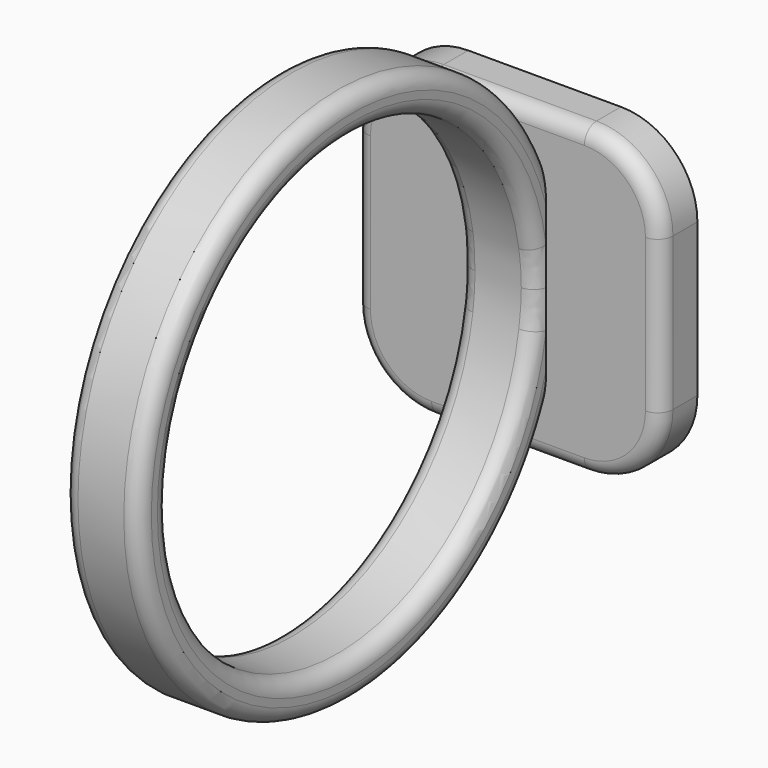
from build123d import *

# Parameters (mm, degrees)
F0_W         = 20
F0_H         = 20
F1_DEPTH     = 3
F2_R         = 17.5
F2_R_2       = 15
F3_DEPTH     = 2.5
F4_R         = 1
F5_T1_DEPTH  = 15.5
F5_T4_ANGLE  = 90
F5_T6_ANGLE  = 90
F5_T8_ANGLE  = 90
F5_T10_ANGLE = 90


# Not quite as in the source:
# - a fillet or chamfer that OpenCascade refuses, or shapes differently, is made with other operations: its cross-section is extruded or revolved along the edge and cut away or added


with BuildPart() as f1:
    # F0 (on Front) → F1 (new body)
    with BuildSketch(Plane.XZ):
        Rectangle(F0_W, F0_H)
    extrude(amount=F1_DEPTH)

    # F2 (on Right) → F3 (join, symmetric)
    with BuildSketch(Plane.YZ):
        with Locations((-18.8078675419, 0)):
            Circle(F2_R)
        with Locations((-18.8078675419, 0)):
            Circle(F2_R_2, mode=Mode.SUBTRACT)
    extrude(amount=F3_DEPTH, both=True)

    # F4 (call 1 of 5: OpenCascade refuses the feature's edges together)
    f4_edges = [f1.edges().sort_by_distance(p)[0] for p in [
        (2.5, -36.307868, 0),
    ]]
    fillet(f4_edges, radius=F4_R)

    # F4#2 (call 2 of 5)
    f4_2_edges = [f1.edges().sort_by_distance(p)[0] for p in [
        (-2.5, -36.307868, 0),
    ]]
    fillet(f4_2_edges, radius=F4_R)

    # F4#3 (call 3 of 5)
    f4_3_edges = [f1.edges().sort_by_distance(p)[0] for p in [
        (-2.5, -33.807868, 0),
    ]]
    fillet(f4_3_edges, radius=F4_R)

    # F4#4 (call 4 of 5)
    f4_4_edges = [f1.edges().sort_by_distance(p)[0] for p in [
        (2.5, -33.807868, 0),
    ]]
    fillet(f4_4_edges, radius=F4_R)

    # F4#5 (call 5 of 5)
    f4_5_edges = [f1.edges().sort_by_distance(p)[0] for p in [
        (10, -3, 0),
        (0, -3, 10),
        (-10, -3, 0),
        (0, -3, -10),
    ]]
    fillet(f4_5_edges, radius=F4_R)

    # F5: fillet of radius 5 on 4 edges, made by hand

    # F5_s2 → F5_t1 (cut)
    with BuildSketch(Plane.XZ.offset(-12.5)):
        with BuildLine():
            ThreePointArc((-5, 10), (-8.5355339059, 8.5355339059), (-10, 5))
            Line((-10, 5), (-10, 10))
            Line((-10, 10), (-5, 10))
        make_face()
        with BuildLine():
            ThreePointArc((-5, -10), (-8.5355339059, -8.5355339059), (-10, -5))
            Line((-10, -5), (-10, -10))
            Line((-10, -10), (-5, -10))
        make_face()
        with BuildLine():
            ThreePointArc((10, 5), (8.5355339059, 8.5355339059), (5, 10))
            Line((5, 10), (10, 10))
            Line((10, 10), (10, 5))
        make_face()
        with BuildLine():
            ThreePointArc((10, -5), (8.5355339059, -8.5355339059), (5, -10))
            Line((5, -10), (10, -10))
            Line((10, -10), (10, -5))
        make_face()
    extrude(amount=F5_T1_DEPTH, mode=Mode.SUBTRACT)

    # F5_s3 → F5_t4 (revolve, cut)
    with BuildSketch(Plane.YZ.offset(5)):
        with BuildLine():
            ThreePointArc((-3, -9), (-2.7071067812, -9.7071067812), (-2, -10))
            Line((-2, -10), (-3, -10))
            Line((-3, -10), (-3, -9))
        make_face()
    revolve(axis=Axis((5, -3, -5), (0, -1, 0)), revolution_arc=F5_T4_ANGLE, mode=Mode.SUBTRACT)

    # F5_s5 → F5_t6 (revolve, cut)
    with BuildSketch(Plane.XY.offset(5)):
        with BuildLine():
            ThreePointArc((9, -3), (9.7071067812, -2.7071067812), (10, -2))
            Line((10, -2), (10, -3))
            Line((10, -3), (9, -3))
        make_face()
    revolve(axis=Axis((5, -3, 5), (0, -1, 0)), revolution_arc=F5_T6_ANGLE, mode=Mode.SUBTRACT)

    # F5_s7 → F5_t8 (revolve, cut)
    with BuildSketch(Plane.XY.offset(-5)):
        with BuildLine():
            ThreePointArc((-9, -3), (-9.7071067812, -2.7071067812), (-10, -2))
            Line((-10, -2), (-10, -3))
            Line((-10, -3), (-9, -3))
        make_face()
    revolve(axis=Axis((-5, -3, -5), (0, -1, 0)), revolution_arc=F5_T8_ANGLE, mode=Mode.SUBTRACT)

    # F5_s9 → F5_t10 (revolve, cut)
    with BuildSketch(Plane.YZ.offset(-5)):
        with BuildLine():
            ThreePointArc((-3, 9), (-2.7071067812, 9.7071067812), (-2, 10))
            Line((-2, 10), (-3, 10))
            Line((-3, 10), (-3, 9))
        make_face()
    revolve(axis=Axis((-5, -3, 5), (0, -1, 0)), revolution_arc=F5_T10_ANGLE, mode=Mode.SUBTRACT)


solid = f1.part
